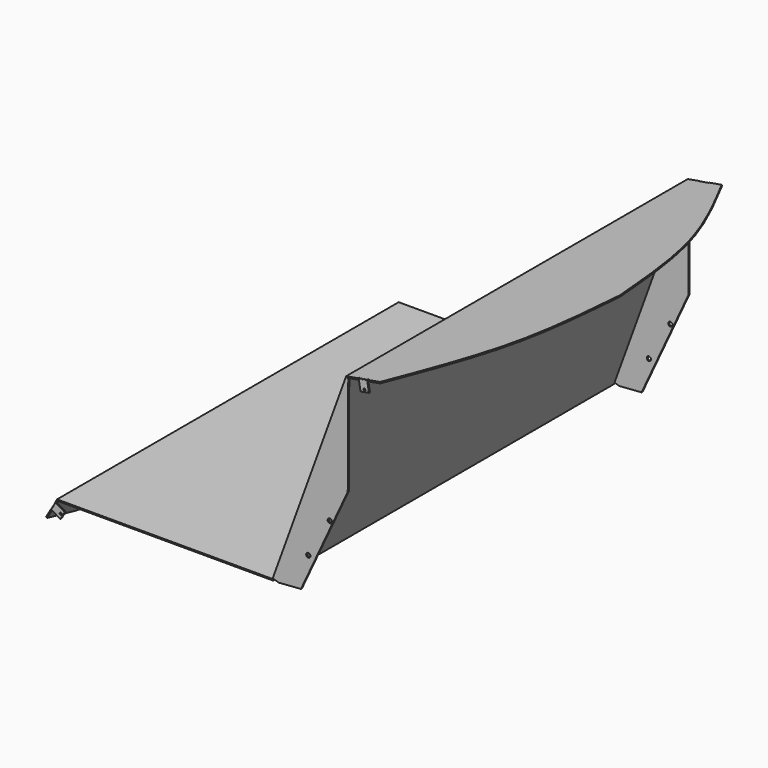
from build123d import *

# Parameters (mm, degrees)
F1_DEPTH  = 500
F3_DEPTH  = 25
F5_DEPTH  = 25
F6_W      = 3
F6_H      = 22
F7_DEPTH  = 25
F8_W      = 22
F8_H      = 3
F9_DEPTH  = 25
F11_DEPTH = 3
F12_R     = 1.5
F13_R     = 2.5
F14_DEPTH = 25
F16_DEPTH = 3
F17_R     = 1.5
F18_R     = 2.5
F19_DEPTH = 25
F20_W     = 3
F20_H     = 502.47
F21_DEPTH = 25
F23_DEPTH = 3
F24_R     = 5
F25_DEPTH = 25


with BuildPart() as f1:
    # F0 (on Front) → F1 (new body)
    with BuildSketch(Plane.XZ):
        Polygon((504.47, 0), (0, 0), (-81.595, -141.3266856436), (-78.9969237661, -142.8266856566), (1.7320508226, -3.0000000261), (506.5706226329, -3.0000000261), (679.2355833198, 471.3930805921), (919.3296938381, 513.7281501857), (918.8087493006, 516.6825734704), (677.0089017035, 474.0467364079), align=None)
    extrude(amount=F1_DEPTH)

    # F2 (on face) → F3 (cut)
    with BuildSketch(Plane(origin=(0, 0, 0), x_dir=(0, -1, 0), z_dir=(-0.8660254038, 0, 0.5))):
        with BuildLine():
            add(Edge.make_bspline(
                [(0, -163.19), (92.9037991034, -155.737461166), (273.0256641206, -141.2884805339), (425.9509699186, -80.7188457637), (500, -51.39)],
                knots=[0, 0, 0, 0, 0.5157830178, 1, 1, 1, 1], degree=3))
            Line((0, -163.19), (0, -174.6820956469))
            Line((0, -174.6820956469), (528.7734270096, -174.6820956469))
            Line((528.7734270096, -174.6820956469), (528.7734270096, -51.39))
            Line((528.7734270096, -51.39), (500, -51.39))
        make_face()
    extrude(amount=-F3_DEPTH, mode=Mode.SUBTRACT)

    # F4 (on face) → F5 (cut)
    with BuildSketch(Plane(origin=(-60.6524500815, 0, 343.9771374623), x_dir=(0.984807753, 0, 0.1736481777), z_dir=(-0.1736481777, 0, 0.984807753))):
        with BuildLine():
            Line((994.5709671621, -500), (994.5709671621, 0))
            add(Edge.make_bspline(
                [(994.5709671621, 0), (985.1762808521, -87.1032361942), (966.2104639681, -262.9456191283), (875.4987714572, -420.4933030834), (829.7209671621, -500)],
                knots=[0, 0, 0, 0, 0.4953483611, 1, 1, 1, 1], degree=3))
            Line((829.7209671621, -500), (994.5709671621, -500))
        make_face()
    extrude(amount=-F5_DEPTH, mode=Mode.SUBTRACT)

    # F6 (on face) → F7 (cut)
    with BuildSketch(Plane(origin=(0, 0, 0), x_dir=(0, -1, 0), z_dir=(-0.8660254038, 0, 0.5))):
        with Locations((498.5, -19)):
            Rectangle(F6_W, F6_H)
    extrude(amount=-F7_DEPTH, mode=Mode.SUBTRACT)

    # F8 (on face) → F9 (cut)
    with BuildSketch(Plane(origin=(-60.6524500815, 0, 343.9771374623), x_dir=(0.984807753, 0, 0.1736481777), z_dir=(-0.1736481777, 0, 0.984807753))):
        with Locations((788.6809671621, -498.5)):
            Rectangle(F8_W, F8_H)
    extrude(amount=-F9_DEPTH, mode=Mode.SUBTRACT)

    # F10 (on face) → F11 (join)
    with BuildSketch(Plane.XZ.offset(497)):
        Polygon((730.4443408179, 456.8646688183), (725.894758563, 482.6666319473), (706.1986035028, 479.1936683939), (710.7481857577, 453.391705265), align=None)
    extrude(amount=F11_DEPTH)

    # F12
    f12_edges = [f1.edges().sort_by_distance(p)[0] for p in [
        (716.046681, -500, 480.93015),
        (716.567626, -497, 477.975727),
    ]]
    fillet(f12_edges, radius=F12_R)

    # F13 (on face) → F14 (cut)
    with BuildSketch(Plane.XZ.offset(500)):
        with Locations((719.7280223994, 460.0522258067)):
            Circle(F13_R)
    extrude(amount=-F14_DEPTH, mode=Mode.SUBTRACT)

    # F15 (on face) → F16 (join)
    with BuildSketch(Plane.XZ.offset(497)):
        Polygon((-4.5, -7.7942286341), (-14.5, -25.1147367097), (8.0339810065, -38.1247367097), (18.0339810065, -20.8042286341), align=None)
    extrude(amount=F16_DEPTH)

    # F17
    f17_edges = [f1.edges().sort_by_distance(p)[0] for p in [
        (-9.5, -500, -16.454483),
        (-6.901924, -497, -17.954483),
    ]]
    fillet(f17_edges, radius=F17_R)

    # F18 (on face) → F19 (cut)
    with BuildSketch(Plane.XZ.offset(500)):
        with Locations((8.7038539875, -26.9644826719)):
            Circle(F18_R)
    extrude(amount=-F19_DEPTH, mode=Mode.SUBTRACT)

    # F20 (on face) → F21 (cut)
    with BuildSketch(Plane(origin=(445.4582201101, 0, -162.1335327293), x_dir=(0, -1, 0), z_dir=(-0.9396926208, 0, 0.3420201433))):
        with Locations((498.5, 424.7739017035)):
            Rectangle(F20_W, F20_H)
    extrude(amount=-F21_DEPTH, mode=Mode.SUBTRACT)

    # F22 (on face) → F23 (join)
    with BuildSketch(Plane.XZ.offset(497)):
        Polygon((679.1439393037, 471.1412907274), (676.3248614168, 472.1673511663), (505.1540402867, 1.8793852416), (507.9731181735, 0.8533248027), align=None)
        Polygon((681.9630171416, 470.1152303063), (679.1439393037, 471.1412907274), (507.9731181735, 0.8533248027), (518.281546199, -2.8986361607), (571.1954295904, 0.9396926208), (680.732997499, 236.8955152162), align=None)
    extrude(amount=F23_DEPTH)

    # F24 (on face) → F25 (cut)
    with BuildSketch(Plane.XZ.offset(500)):
        with Locations((588.350177503, 75.9943071688)):
            Circle(F24_R)
        with Locations((638.6515103983, 163.4973151683)):
            Circle(F24_R)
    extrude(amount=-F25_DEPTH, mode=Mode.SUBTRACT)

    # F26: F1 across face


with BuildPart() as f1_1:
    add(f1.part)
    add(f1.part.mirror(Plane(origin=(434.4998955086, 0, 160.5222009708), x_dir=(1, 0, 0), z_dir=(0, 1, 0))))


solid = f1_1.part
